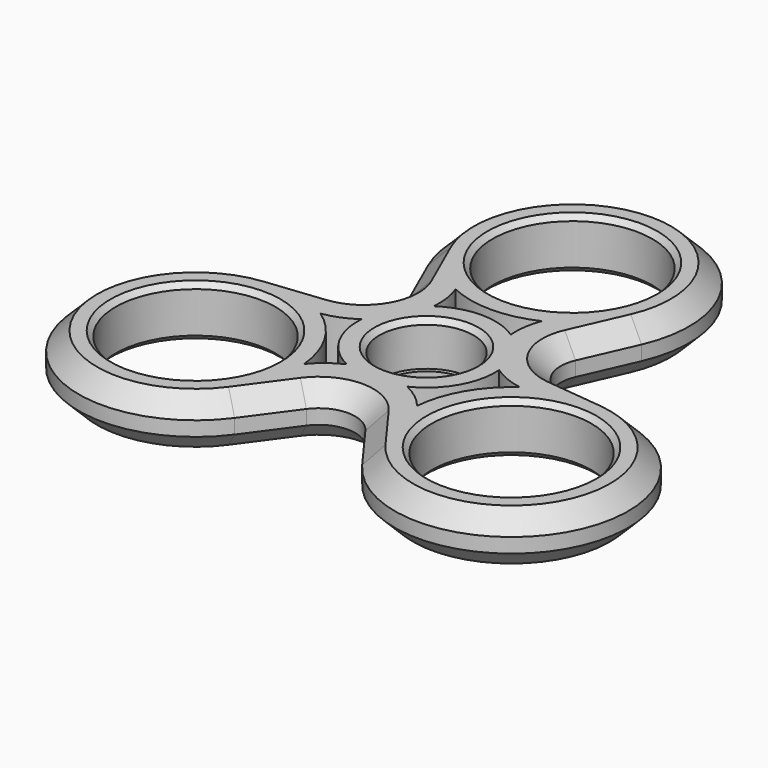
from build123d import *

# Parameters (mm, degrees)
F0_R     = 10.95
F0_R_2   = 6.45
F1_DEPTH = 7
F2_R     = 5
F3_SIZE  = 2.5
F4_R     = 6.45
F4_R_2   = 5.85
F5_DEPTH = 1
F6_SIZE  = 0.7
F8_DEPTH = 25


with BuildPart() as f1:
    # F0 (on Top) → F1 (new body)
    with BuildSketch(Plane.XY):
        with BuildLine():
            Line((8.6602540378, 5), (14.6370370137, 18.538022945))
            ThreePointArc((14.6370370137, 18.538022945), (0, 41), (-14.6370370137, 18.538022945))
            Line((-14.6370370137, 18.538022945), (-8.6602540378, 5))
            Line((-8.6602540378, 5), (-23.3729173132, 3.4070344175))
            ThreePointArc((-23.3729173132, 3.4070344175), (-35.5070415552, -20.5), (-8.7358802995, -21.9450573625))
            Line((-8.7358802995, -21.9450573625), (0, -10))
            Line((0, -10), (8.7358802995, -21.9450573625))
            ThreePointArc((8.7358802995, -21.9450573625), (35.5070415552, -20.5), (23.3729173132, 3.4070344175))
            Line((23.3729173132, 3.4070344175), (8.6602540378, 5))
        make_face()
        with Locations((-21.6506350946, -12.5)):
            Circle(F0_R, mode=Mode.SUBTRACT)
        with Locations((21.6506350946, -12.5)):
            Circle(F0_R, mode=Mode.SUBTRACT)
        Circle(F0_R_2, mode=Mode.SUBTRACT)
        with Locations((0, 25)):
            Circle(F0_R, mode=Mode.SUBTRACT)
    extrude(amount=F1_DEPTH)

    # F2
    f2_edges = [f1.edges().sort_by_distance(p)[0] for p in [
        (0, -10, 3.5),
        (8.660254, 5, 3.5),
        (-8.660254, 5, 3.5),
    ]]
    fillet(f2_edges, radius=F2_R)

    # F3
    f3_edges = [f1.edges().sort_by_distance(p)[0] for p in [
        (-19.415113, 3.835553, 7),
        (-6.385871, -18.731758, 0),
        (19.415113, 3.835553, 0),
        (19.415113, 3.835553, 7),
        (11.665396, 6.735019, 0),
        (35.507042, -20.5, 0),
        (13.029243, 14.896205, 0),
        (6.385871, -18.731758, 0),
        (0, 41, 0),
        (0, -13.470039, 0),
        (-13.029243, 14.896205, 0),
        (-11.665396, 6.735019, 0),
        (-35.507042, -20.5, 0),
        (-19.415113, 3.835553, 0),
        (11.665396, 6.735019, 7),
        (35.507042, -20.5, 7),
        (13.029243, 14.896205, 7),
        (6.385871, -18.731758, 7),
        (0, 41, 7),
        (0, -13.470039, 7),
        (-13.029243, 14.896205, 7),
        (-6.385871, -18.731758, 7),
        (-11.665396, 6.735019, 7),
        (-35.507042, -20.5, 7),
    ]]
    chamfer(f3_edges, length=F3_SIZE)

    # F4 (on face) → F5 (join)
    with BuildSketch(Plane(origin=(0, 0, 0), x_dir=(1, 0, 0), z_dir=(0, 0, -1))):
        Circle(F4_R)
        Circle(F4_R_2, mode=Mode.SUBTRACT)
    extrude(amount=-F5_DEPTH)

    # F6
    f6_edges = [f1.edges().sort_by_distance(p)[0] for p in [
        (-6.45, 0, 7),
        (-32.600635, -12.5, 7),
        (10.700635, -12.5, 7),
        (-10.95, 25, 7),
        (-32.600635, -12.5, 0),
        (10.700635, -12.5, 0),
        (-10.95, 25, 0),
    ]]
    chamfer(f6_edges, length=F6_SIZE)

    # F7 (on face) → F8 (cut)
    with BuildSketch(Plane.XY.offset(7)):
        with BuildLine():
            ThreePointArc((-4.1486247409, -8.4906662141), (-8.1839400658, -4.725), (-9.4274450069, 0.6525186907))
            ThreePointArc((-9.4274450069, 0.6525186907), (-11.4491842198, -0.4430009845), (-13.6635486442, -1.0628259595))
            ThreePointArc((-13.6635486442, -1.0628259595), (-9.5695807118, -5.525), (-7.7522086028, -11.3015672519))
            ThreePointArc((-7.7522086028, -11.3015672519), (-6.1082422164, -9.6937838947), (-4.1486247409, -8.4906662141))
        make_face()
        with BuildLine():
            ThreePointArc((-5.278820266, 7.8381475234), (0, 9.45), (5.278820266, 7.8381475234))
            ThreePointArc((5.278820266, 7.8381475234), (5.3409420034, 10.1367848792), (5.9113400414, 12.3643932114))
            ThreePointArc((5.9113400414, 12.3643932114), (0, 11.05), (-5.9113400414, 12.3643932114))
            ThreePointArc((-5.9113400414, 12.3643932114), (-5.3409420034, 10.1367848792), (-5.278820266, 7.8381475234))
        make_face()
        with BuildLine():
            ThreePointArc((9.4274450069, 0.6525186907), (8.1839400658, -4.725), (4.1486247409, -8.4906662141))
            ThreePointArc((4.1486247409, -8.4906662141), (6.1082422164, -9.6937838947), (7.7522086028, -11.3015672519))
            ThreePointArc((7.7522086028, -11.3015672519), (9.5695807118, -5.525), (13.6635486442, -1.0628259595))
            ThreePointArc((13.6635486442, -1.0628259595), (11.4491842198, -0.4430009845), (9.4274450069, 0.6525186907))
        make_face()
    extrude(amount=-F8_DEPTH, mode=Mode.SUBTRACT)


solid = f1.part
